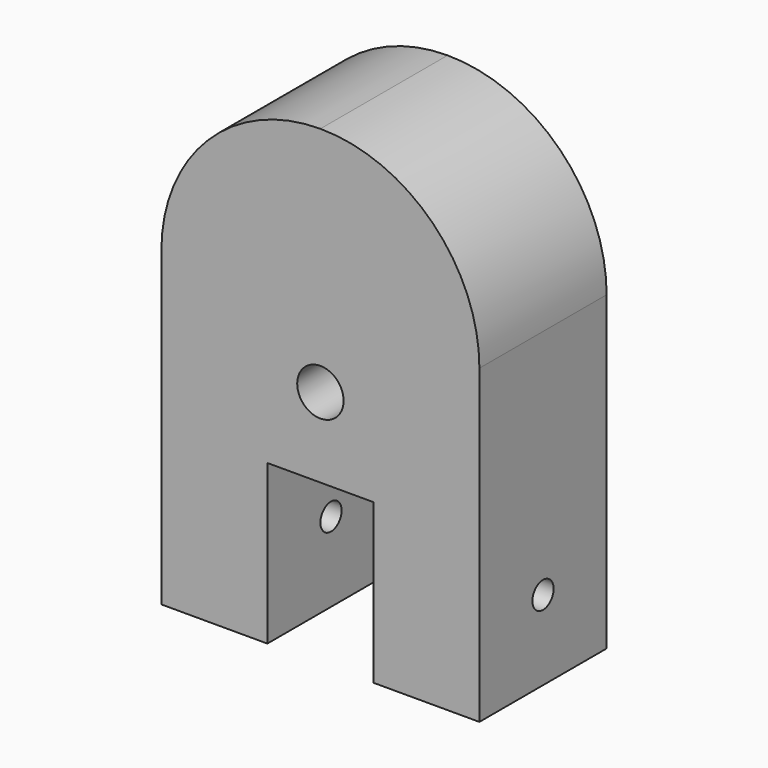
from build123d import *

# Parameters (mm, degrees)
F1_DEPTH = 76.2
F2_R     = 76.19999
F4_D     = 22.225
F6_D     = 12.7


# Not quite as in the source:
# - a fillet or chamfer is up to 0.001 mm smaller than in the source, because OpenCascade refuses the exact size


with BuildPart() as f1:
    # F0 (on Front) → F1 (new body)
    with BuildSketch(Plane.XZ):
        Polygon((-50.8, 0), (0, 0), (0, 76.2), (50.8, 76.2), (50.8, 0), (101.6, 0), (101.6, 225.425), (-50.8, 225.425), align=None)
    extrude(amount=F1_DEPTH)

    # F2 (radius 76.2 in the source; OpenCascade refuses exactly that, so slightly less here)
    f2_edges = [f1.edges().sort_by_distance(p)[0] for p in [
        (101.6, -38.1, 225.425),
        (-50.8, -38.1, 225.425),
    ]]
    fillet(f2_edges, radius=F2_R)

    # F4 (through all)
    with Locations(Plane.XZ.offset(76.2)):
        with Locations((25.4, 114.3)):
            Hole(F4_D / 2)

    # F6 (through all)
    with Locations(Plane.YZ.offset(101.6)):
        with Locations((-38.1, 38.1)):
            Hole(F6_D / 2)


solid = f1.part
